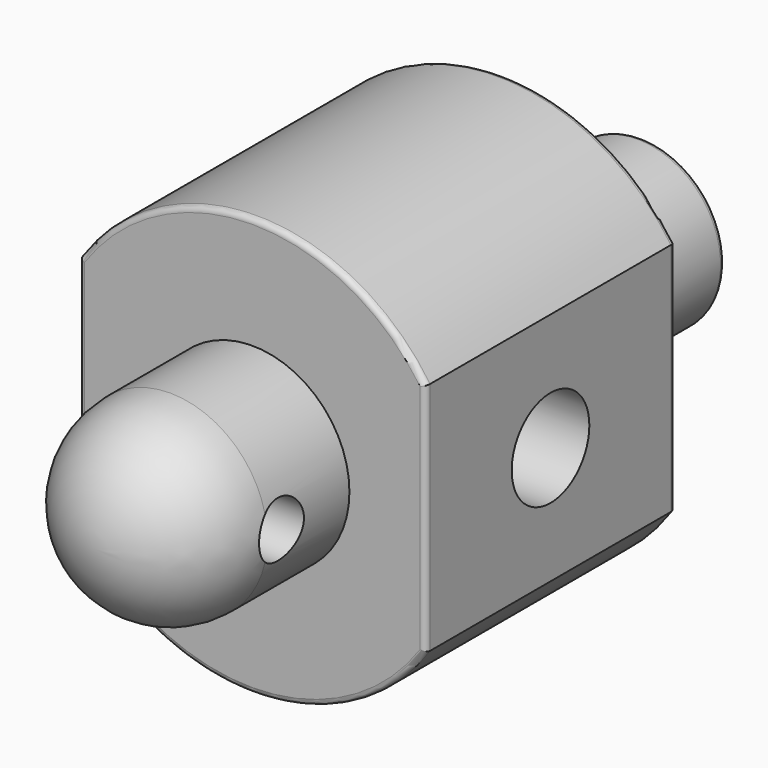
from build123d import *

# Parameters (mm, degrees)
F1_DEPTH = 11.25
F2_R     = 1.75
F3_DEPTH = 15
F4_R     = 3
F5_DEPTH = 6.3
F6_R     = 3.5
F7_DEPTH = 7.2
F8_R     = 1
F9_DEPTH = 15
F11_R    = 0.2


# Not quite as in the source:
# - a fillet or chamfer that OpenCascade refuses, or shapes differently, is made with other operations: its cross-section is extruded or revolved along the edge and cut away or added


with BuildPart() as f1:
    # F0 (on Front) → F1 (new body)
    with BuildSketch(Plane.XZ):
        with BuildLine():
            Line((6.25, 0), (6.25, 4.2355637169))
            ThreePointArc((6.25, 4.2355637169), (0, 7.55), (-6.25, 4.2355637169))
            Line((-6.25, 4.2355637169), (-6.25, -4.2355637169))
            ThreePointArc((-6.25, -4.2355637169), (0, -7.55), (6.25, -4.2355637169))
            Line((6.25, -4.2355637169), (6.25, 0))
        make_face()
    extrude(amount=F1_DEPTH)

    # F2 (on face) → F3 (cut)
    with BuildSketch(Plane.YZ.offset(6.25)):
        with Locations((-5.625, 0)):
            Circle(F2_R)
    extrude(amount=-F3_DEPTH, mode=Mode.SUBTRACT)

    # F4 (on face) → F5 (join)
    with BuildSketch(Plane(origin=(0, 0, 0), x_dir=(-1, 0, 0), z_dir=(0, 1, 0))):
        Circle(F4_R)
    extrude(amount=F5_DEPTH)

    # F6 (on face) → F7 (join)
    with BuildSketch(Plane.XZ.offset(11.25)):
        Circle(F6_R)
    extrude(amount=F7_DEPTH)

    # F8 (on face) → F9 (cut)
    with BuildSketch(Plane.YZ.offset(6.25)):
        with Locations((-14.3, 0)):
            Circle(F8_R)
    extrude(amount=-F9_DEPTH, mode=Mode.SUBTRACT)

    # F10: fillet of radius 3.5 on 1 edges, made by hand

    # F10_s1 → F10_t2 (revolve, cut)
    with BuildSketch(Plane.XY):
        with BuildLine():
            ThreePointArc((3.5, -14.95), (2.4748737342, -17.4248737342), (0, -18.45))
            Line((0, -18.45), (3.5, -18.45))
            Line((3.5, -18.45), (3.5, -14.95))
        make_face()
    revolve(axis=Axis((0, -18.45, 0), (0, -1, 0)), mode=Mode.SUBTRACT)

    # F11
    f11_edges = [f1.edges().sort_by_distance(p)[0] for p in [
        (3, 6.3, 0),
        (0, 0, 7.55),
        (6.25, 0, 0),
        (0, 0, -7.55),
        (-6.25, 0, 0),
        (0, -11.25, 7.55),
        (0, -11.25, -7.55),
        (-6.25, -11.25, 0),
        (6.25, -11.25, 0),
    ]]
    fillet(f11_edges, radius=F11_R)


solid = f1.part
